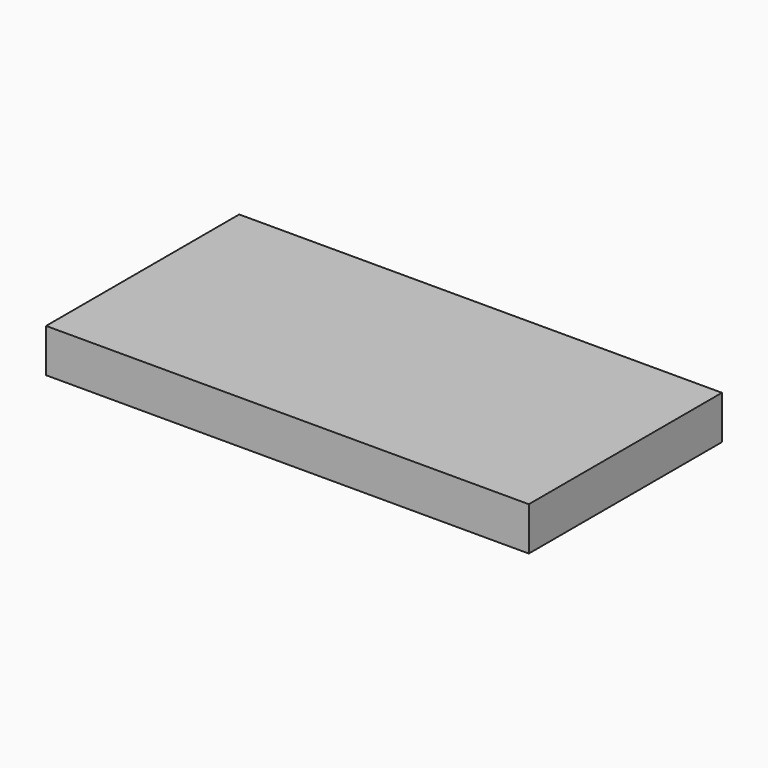
from build123d import *

# Parameters (mm, degrees)
F0_W         = 100
F0_H         = 50
F1_DEPTH     = 3
F2_W         = 100
F2_H         = 50
F3_TEXT_SIZE = 45.3538843122
F4_DEPTH     = 2
F5_DEPTH     = 2
F6_DEPTH     = 2
F4_FACE_W    = 100
F4_FACE_H    = 50
F7_DEPTH     = 2
F7_FACE_W    = 100
F7_FACE_H    = 50
F8_DEPTH     = 2


# Not quite as in the source:
# - Text() gives the source's letters only with a copy of the font that has no kerning and outlines rounded to 1/6400 em; it was checked with that copy


with BuildPart() as f1:
    # F0 (on Top) → F1 (new body)
    with BuildSketch(Plane.XY):
        with Locations((-50, 25)):
            Rectangle(F0_W, F0_H)
    extrude(amount=F1_DEPTH)

    # F2 (on face) + F3 (on face) → F4 (join)
    with BuildSketch(Plane.XY.offset(3)):
        with Locations((-50, 25)):
            Rectangle(F2_W, F2_H)
    with BuildSketch(Plane.XY.offset(3)):
        with Locations((-91.4267910924, 7.3682615957)):
            Text('Ella', F3_TEXT_SIZE, font='Noto Sans', font_style=FontStyle.BOLD, text_align=(TextAlign.LEFT, TextAlign.BOTTOM))
    extrude(amount=F4_DEPTH)

    # F3 (on face) → F5 (join)
    with BuildSketch(Plane.XY.offset(3)):
        with Locations((-91.4267910924, 7.3682615957)):
            Text('Ella', F3_TEXT_SIZE, font='Noto Sans', font_style=FontStyle.BOLD, text_align=(TextAlign.LEFT, TextAlign.BOTTOM))
    extrude(amount=F5_DEPTH)

    # F3 (on face) → F6 (join)
    with BuildSketch(Plane.XY.offset(3)):
        with Locations((-91.4267910924, 7.3682615957)):
            Text('Ella', F3_TEXT_SIZE, font='Noto Sans', font_style=FontStyle.BOLD, text_align=(TextAlign.LEFT, TextAlign.BOTTOM))
    extrude(amount=F6_DEPTH)

    # F3 (on face) + F4_face (on face) → F7 (join)
    with BuildSketch(Plane.XY.offset(3)):
        with Locations((-91.4267910924, 7.3682615957)):
            Text('Ella', F3_TEXT_SIZE, font='Noto Sans', font_style=FontStyle.BOLD, text_align=(TextAlign.LEFT, TextAlign.BOTTOM))
    with BuildSketch(Plane(origin=(-50, 25, 5), x_dir=(1, 0, 0), z_dir=(0, 0, 1))):
        Rectangle(F4_FACE_W, F4_FACE_H)
    extrude(amount=F7_DEPTH)

    # F3 (on face) + F7_face (on face) → F8 (join)
    with BuildSketch(Plane.XY.offset(3)):
        with Locations((-91.4267910924, 7.3682615957)):
            Text('Ella', F3_TEXT_SIZE, font='Noto Sans', font_style=FontStyle.BOLD, text_align=(TextAlign.LEFT, TextAlign.BOTTOM))
    with BuildSketch(Plane(origin=(-50, 25, 7), x_dir=(1, 0, 0), z_dir=(0, 0, 1))):
        Rectangle(F7_FACE_W, F7_FACE_H)
    extrude(amount=F8_DEPTH)


solid = f1.part
